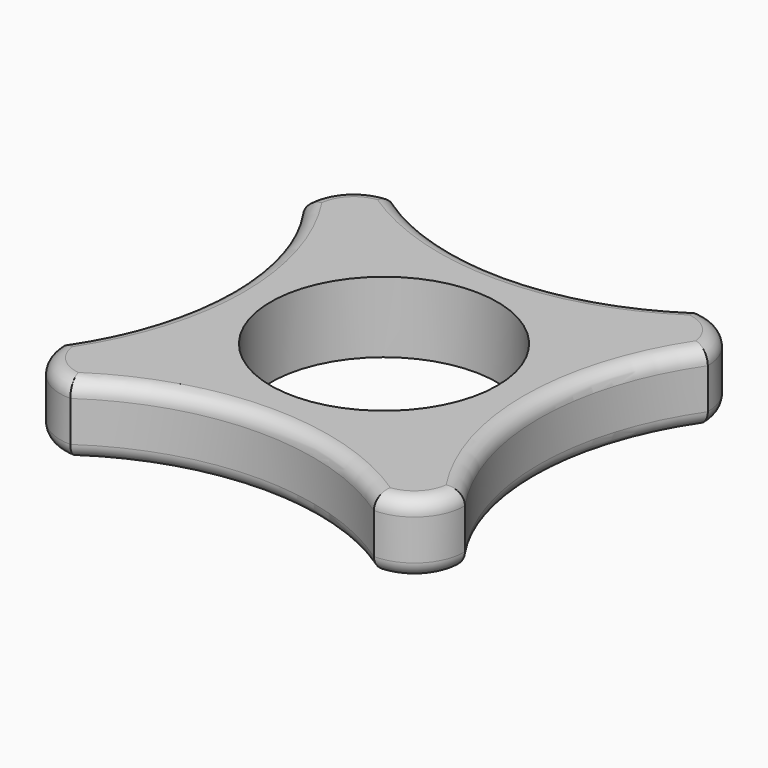
from build123d import *

# Parameters (mm, degrees)
F0_R         = 11.2
F1_DEPTH     = 7
F2_T3_ANGLE  = 85.2645116728
F2_T6_ANGLE  = 175.9781935424
F2_T9_ANGLE  = 85.2645116728
F2_T12_ANGLE = 175.9781935424
F2_T15_ANGLE = 85.2645116728
F2_T18_ANGLE = 175.9781935424
F2_T21_ANGLE = 85.2645116728
F2_T24_ANGLE = 175.9781935424
F3_T2_ANGLE  = 85.2645116728
F3_T4_ANGLE  = 85.2645116728
F3_T6_ANGLE  = 85.2645116728
F3_T8_ANGLE  = 85.2645116728
F3_T10_ANGLE = 175.9781935424
F3_T12_ANGLE = 175.9781935424
F3_T14_ANGLE = 175.9781935424
F3_T16_ANGLE = 175.9781935424


# Not quite as in the source:
# - a fillet or chamfer that OpenCascade refuses, or shapes differently, is made with other operations: its cross-section is extruded or revolved along the edge and cut away or added


with BuildPart() as f1:
    # F0 (on Top) → F1 (new body)
    with BuildSketch(Plane.XY):
        with BuildLine():
            ThreePointArc((15, 20), (0, 15.3403332466), (-15, 20))
            ThreePointArc((-15, 20), (-18.5355339059, 18.5355339059), (-20, 15))
            ThreePointArc((-20, 15), (-15.3403332466, 0), (-20, -15))
            ThreePointArc((-20, -15), (-18.5355339059, -18.5355339059), (-15, -20))
            ThreePointArc((-15, -20), (0, -15.3403332466), (15, -20))
            ThreePointArc((15, -20), (18.5355339059, -18.5355339059), (20, -15))
            ThreePointArc((20, -15), (15.3403332466, 0), (20, 15))
            ThreePointArc((20, 15), (18.5355339059, 18.5355339059), (15, 20))
        make_face()
        Circle(F0_R, mode=Mode.SUBTRACT)
    extrude(amount=F1_DEPTH)

    # F2: fillet of radius 1.5 on 8 edges, made by hand


with BuildPart() as f2_tool1:
    # F2_s2 → F2_t3 (revolve)
    with BuildSketch(Plane(origin=(20.8353956291, 19.1807876052, 0), x_dir=(0, 0, 1), z_dir=(0.7357159093, 0.6772902634, 0))):
        with BuildLine():
            ThreePointArc((5.5, -4.2896840575), (6.5606601718, -3.8503442293), (7, -2.7896840575))
            Line((7, -2.7896840575), (7, -4.2896840575))
            Line((7, -4.2896840575), (5.5, -4.2896840575))
        make_face()
    revolve(axis=Axis((0, 41.8135240681, 7), (0, 0, -1)), revolution_arc=F2_T3_ANGLE)


with BuildPart() as f2_tool4:
    # F2_s5 → F2_t6 (revolve)
    with BuildSketch(Plane(origin=(14.4555096977, 15.5075517385, 0), x_dir=(0, 0, 1), z_dir=(-0.6818591731, -0.7314834708, 0))):
        with BuildLine():
            ThreePointArc((5.5, -5.7443644649), (6.5606601718, -5.3050246367), (7, -4.2443644649))
            Line((7, -4.2443644649), (7, -5.7443644649))
            Line((7, -5.7443644649), (5.5, -5.7443644649))
        make_face()
    revolve(axis=Axis((15, 15, 7), (0, 0, 1)), revolution_arc=F2_T6_ANGLE)


with BuildPart() as f2_tool7:
    # F2_s8 → F2_t9 (revolve)
    with BuildSketch(Plane(origin=(19.1807876052, -20.8353956291, 0), x_dir=(0, 0, 1), z_dir=(0.6772902634, -0.7357159093, 0))):
        with BuildLine():
            ThreePointArc((5.5, -4.2896840575), (6.5606601718, -3.8503442293), (7, -2.7896840575))
            Line((7, -2.7896840575), (7, -4.2896840575))
            Line((7, -4.2896840575), (5.5, -4.2896840575))
        make_face()
    revolve(axis=Axis((41.8135240681, 0, 7), (0, 0, -1)), revolution_arc=F2_T9_ANGLE)


with BuildPart() as f2_tool10:
    # F2_s11 → F2_t12 (revolve)
    with BuildSketch(Plane(origin=(15.5075517385, -14.4555096977, 0), x_dir=(0, 0, 1), z_dir=(-0.7314834708, 0.6818591731, 0))):
        with BuildLine():
            ThreePointArc((5.5, -5.7443644649), (6.5606601718, -5.3050246367), (7, -4.2443644649))
            Line((7, -4.2443644649), (7, -5.7443644649))
            Line((7, -5.7443644649), (5.5, -5.7443644649))
        make_face()
    revolve(axis=Axis((15, -15, 7), (0, 0, 1)), revolution_arc=F2_T12_ANGLE)


with BuildPart() as f2_tool13:
    # F2_s14 → F2_t15 (revolve)
    with BuildSketch(Plane(origin=(-20.8353956291, -19.1807876052, 0), x_dir=(0, 0, 1), z_dir=(-0.7357159093, -0.6772902634, 0))):
        with BuildLine():
            ThreePointArc((5.5, -4.2896840575), (6.5606601718, -3.8503442293), (7, -2.7896840575))
            Line((7, -2.7896840575), (7, -4.2896840575))
            Line((7, -4.2896840575), (5.5, -4.2896840575))
        make_face()
    revolve(axis=Axis((0, -41.8135240681, 7), (0, 0, -1)), revolution_arc=F2_T15_ANGLE)


with BuildPart() as f2_tool16:
    # F2_s17 → F2_t18 (revolve)
    with BuildSketch(Plane(origin=(-14.4555096977, -15.5075517385, 0), x_dir=(0, 0, 1), z_dir=(0.6818591731, 0.7314834708, 0))):
        with BuildLine():
            ThreePointArc((5.5, -5.7443644649), (6.5606601718, -5.3050246367), (7, -4.2443644649))
            Line((7, -4.2443644649), (7, -5.7443644649))
            Line((7, -5.7443644649), (5.5, -5.7443644649))
        make_face()
    revolve(axis=Axis((-15, -15, 7), (0, 0, 1)), revolution_arc=F2_T18_ANGLE)


with BuildPart() as f2_tool19:
    # F2_s20 → F2_t21 (revolve)
    with BuildSketch(Plane(origin=(-19.1807876052, 20.8353956291, 0), x_dir=(0, 0, 1), z_dir=(-0.6772902634, 0.7357159093, 0))):
        with BuildLine():
            ThreePointArc((5.5, -4.2896840575), (6.5606601718, -3.8503442293), (7, -2.7896840575))
            Line((7, -2.7896840575), (7, -4.2896840575))
            Line((7, -4.2896840575), (5.5, -4.2896840575))
        make_face()
    revolve(axis=Axis((-41.8135240681, 0, 7), (0, 0, -1)), revolution_arc=F2_T21_ANGLE)


with BuildPart() as f2_tool22:
    # F2_s23 → F2_t24 (revolve)
    with BuildSketch(Plane(origin=(-15.5075517385, 14.4555096977, 0), x_dir=(0, 0, 1), z_dir=(0.7314834708, -0.6818591731, 0))):
        with BuildLine():
            ThreePointArc((5.5, -5.7443644649), (6.5606601718, -5.3050246367), (7, -4.2443644649))
            Line((7, -4.2443644649), (7, -5.7443644649))
            Line((7, -5.7443644649), (5.5, -5.7443644649))
        make_face()
    revolve(axis=Axis((-15, 15, 7), (0, 0, 1)), revolution_arc=F2_T24_ANGLE)


with BuildPart() as f1_1:
    add(f1.part)

    # F2_t25: cut F2_tool1, F2_tool4, F2_tool7, F2_tool10, F2_tool13, F2_tool16, F2_tool19, F2_tool22
    add([f2_tool1.part, f2_tool4.part, f2_tool7.part, f2_tool10.part, f2_tool13.part, f2_tool16.part, f2_tool19.part, f2_tool22.part], mode=Mode.SUBTRACT)

    # F3: fillet of radius 1.5 on 8 edges, made by hand

    # F3_s1 → F3_t2 (revolve, cut)
    with BuildSketch(Plane(origin=(-20.8353956291, -19.1807876052, 0), x_dir=(0, 0, 1), z_dir=(-0.7357159093, -0.6772902634, 0))):
        with BuildLine():
            ThreePointArc((0, -2.7896840575), (0.4393398282, -3.8503442293), (1.5, -4.2896840575))
            Line((1.5, -4.2896840575), (0, -4.2896840575))
            Line((0, -4.2896840575), (0, -2.7896840575))
        make_face()
    revolve(axis=Axis((0, -41.8135240681, 0), (0, 0, -1)), revolution_arc=F3_T2_ANGLE, mode=Mode.SUBTRACT)

    # F3_s3 → F3_t4 (revolve, cut)
    with BuildSketch(Plane(origin=(-19.1807876052, 20.8353956291, 0), x_dir=(0, 0, 1), z_dir=(-0.6772902634, 0.7357159093, 0))):
        with BuildLine():
            ThreePointArc((0, -2.7896840575), (0.4393398282, -3.8503442293), (1.5, -4.2896840575))
            Line((1.5, -4.2896840575), (0, -4.2896840575))
            Line((0, -4.2896840575), (0, -2.7896840575))
        make_face()
    revolve(axis=Axis((-41.8135240681, 0, 0), (0, 0, -1)), revolution_arc=F3_T4_ANGLE, mode=Mode.SUBTRACT)

    # F3_s5 → F3_t6 (revolve, cut)
    with BuildSketch(Plane(origin=(20.8353956291, 19.1807876052, 0), x_dir=(0, 0, 1), z_dir=(0.7357159093, 0.6772902634, 0))):
        with BuildLine():
            ThreePointArc((0, -2.7896840575), (0.4393398282, -3.8503442293), (1.5, -4.2896840575))
            Line((1.5, -4.2896840575), (0, -4.2896840575))
            Line((0, -4.2896840575), (0, -2.7896840575))
        make_face()
    revolve(axis=Axis((0, 41.8135240681, 0), (0, 0, -1)), revolution_arc=F3_T6_ANGLE, mode=Mode.SUBTRACT)

    # F3_s7 → F3_t8 (revolve, cut)
    with BuildSketch(Plane(origin=(19.1807876052, -20.8353956291, 0), x_dir=(0, 0, 1), z_dir=(0.6772902634, -0.7357159093, 0))):
        with BuildLine():
            ThreePointArc((0, -2.7896840575), (0.4393398282, -3.8503442293), (1.5, -4.2896840575))
            Line((1.5, -4.2896840575), (0, -4.2896840575))
            Line((0, -4.2896840575), (0, -2.7896840575))
        make_face()
    revolve(axis=Axis((41.8135240681, 0, 0), (0, 0, -1)), revolution_arc=F3_T8_ANGLE, mode=Mode.SUBTRACT)

    # F3_s9 → F3_t10 (revolve, cut)
    with BuildSketch(Plane(origin=(15.5075517385, -14.4555096977, 0), x_dir=(0, 0, 1), z_dir=(-0.7314834708, 0.6818591731, 0))):
        with BuildLine():
            ThreePointArc((0, -4.2443644649), (0.4393398282, -5.3050246367), (1.5, -5.7443644649))
            Line((1.5, -5.7443644649), (0, -5.7443644649))
            Line((0, -5.7443644649), (0, -4.2443644649))
        make_face()
    revolve(axis=Axis((15, -15, 0), (0, 0, 1)), revolution_arc=F3_T10_ANGLE, mode=Mode.SUBTRACT)

    # F3_s11 → F3_t12 (revolve, cut)
    with BuildSketch(Plane(origin=(-14.4555096977, -15.5075517385, 0), x_dir=(0, 0, 1), z_dir=(0.6818591731, 0.7314834708, 0))):
        with BuildLine():
            ThreePointArc((0, -4.2443644649), (0.4393398282, -5.3050246367), (1.5, -5.7443644649))
            Line((1.5, -5.7443644649), (0, -5.7443644649))
            Line((0, -5.7443644649), (0, -4.2443644649))
        make_face()
    revolve(axis=Axis((-15, -15, 0), (0, 0, 1)), revolution_arc=F3_T12_ANGLE, mode=Mode.SUBTRACT)

    # F3_s13 → F3_t14 (revolve, cut)
    with BuildSketch(Plane(origin=(-15.5075517385, 14.4555096977, 0), x_dir=(0, 0, 1), z_dir=(0.7314834708, -0.6818591731, 0))):
        with BuildLine():
            ThreePointArc((0, -4.2443644649), (0.4393398282, -5.3050246367), (1.5, -5.7443644649))
            Line((1.5, -5.7443644649), (0, -5.7443644649))
            Line((0, -5.7443644649), (0, -4.2443644649))
        make_face()
    revolve(axis=Axis((-15, 15, 0), (0, 0, 1)), revolution_arc=F3_T14_ANGLE, mode=Mode.SUBTRACT)

    # F3_s15 → F3_t16 (revolve, cut)
    with BuildSketch(Plane(origin=(14.4555096977, 15.5075517385, 0), x_dir=(0, 0, 1), z_dir=(-0.6818591731, -0.7314834708, 0))):
        with BuildLine():
            ThreePointArc((1.5, -5.7443644649), (0.4393398282, -5.3050246367), (0, -4.2443644649))
            Line((0, -4.2443644649), (0, -5.7443644649))
            Line((0, -5.7443644649), (1.5, -5.7443644649))
        make_face()
    revolve(axis=Axis((15, 15, 0), (0, 0, 1)), revolution_arc=F3_T16_ANGLE, mode=Mode.SUBTRACT)


solid = f1_1.part
